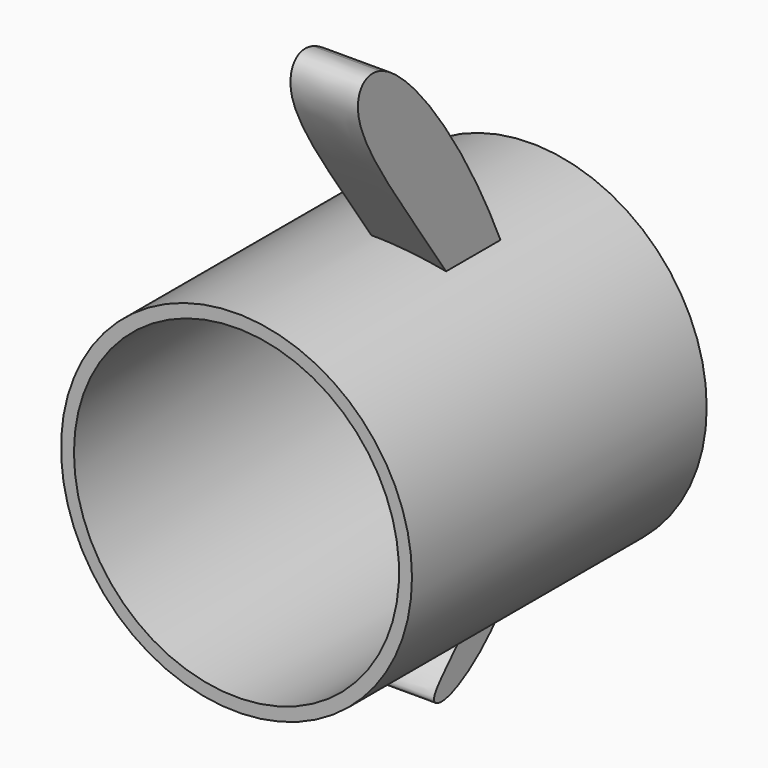
from build123d import *

# Parameters (mm, degrees)
F0_R     = 25
F1_DEPTH = 52.483310923
F4_R     = 23.1594972358
F5_DEPTH = 56.222954765
F7_DEPTH = 9.6091050655


# Not quite as in the source:
# - the program builds the solid bodies; features that only make, move or delete a surface that nothing else refers to are left out


with BuildPart() as f1:
    # F0 (on Front) → F1 (new body)
    with BuildSketch(Plane.XZ):
        Circle(F0_R)
    extrude(amount=-F1_DEPTH)

    # F4 (on face) → F5 (cut)
    with BuildSketch(Plane(origin=(0, 52.483310923, 0), x_dir=(-1, 0, 0), z_dir=(0, 1, 0))):
        Circle(F4_R)
    extrude(amount=-F5_DEPTH, mode=Mode.SUBTRACT)

    # F6 (on Right) → F7 (join)
    with BuildSketch(Plane.YZ):
        with BuildLine():
            add(Edge.make_bspline(
                [(13.5661605746, 52.984289825), (22.7453749365, 49.8663088316), (56.6867603684, -7.723565307), (26.9795580338, -32.0941370462), (20.0288116996, -29.0080395676), (56.4506404561, -5.9541746073), (3.4222546759, 46.2227244929), (10.8831347215, 53.8956557965), (13.5661605746, 52.984289825)],
                knots=[0, 0, 0, 0, 0.2662310005, 0.4435228486, 0.4925757944, 0.6637410127, 0.9221823754, 1, 1, 1, 1], degree=3))
        make_face()
    extrude(amount=F7_DEPTH)


solid = f1.part
